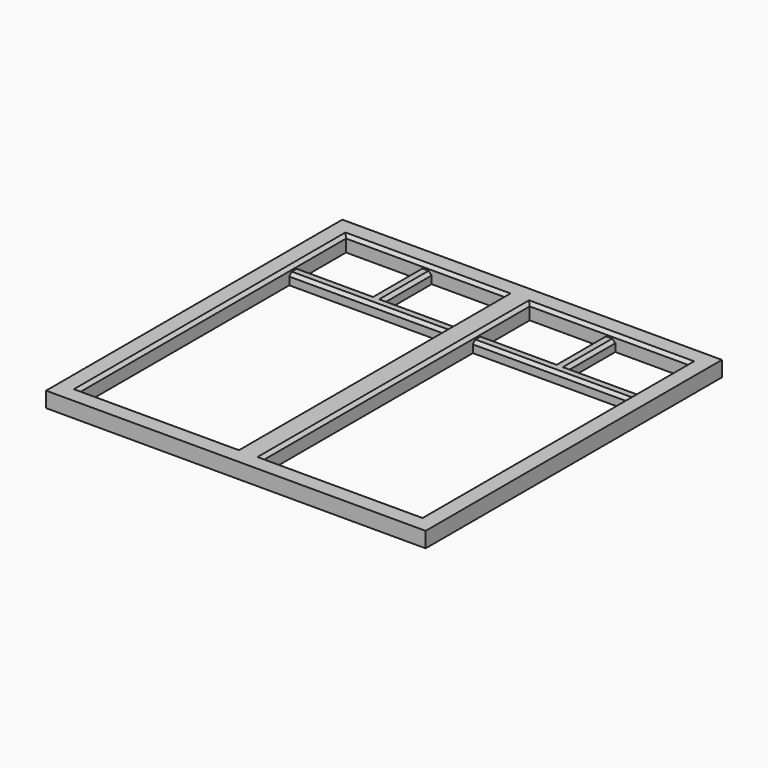
from build123d import *

# Parameters (mm, degrees)
F0_W      = 1230
F0_H      = 1200
F1_DEPTH  = 50
F2_DEPTH  = 35
F3_SIZE   = 10
F3_2_SIZE = 10
F3_3_SIZE = 10


with BuildPart() as f1:
    # F0 (on Top) → F1 (new body)
    with BuildSketch(Plane.XY):
        with Locations((220.3141621128, 45.2047318473)):
            Rectangle(F0_W, F0_H)
        Polygon((-334.6858378872, -494.7952681527), (-334.6858378872, 355.2047318473), (-334.6858378872, 395.2047318473), (-334.6858378872, 585.2047318473), (-97.1858378872, 585.2047318473), (-57.1858378872, 585.2047318473), (180.3141621128, 585.2047318473), (180.3141621128, 395.2047318473), (180.3141621128, 355.2047318473), (180.3141621128, -494.7952681527), align=None, mode=Mode.SUBTRACT)
        Polygon((260.3141621128, -494.7952681527), (260.3141621128, 355.2047318473), (260.3141621128, 395.2047318473), (260.3141621128, 585.2047318473), (497.8141621128, 585.2047318473), (537.8141621128, 585.2047318473), (775.3141621128, 585.2047318473), (775.3141621128, 395.2047318473), (775.3141621128, 355.2047318473), (775.3141621128, -494.7952681527), align=None, mode=Mode.SUBTRACT)
    extrude(amount=F1_DEPTH)

    # F3
    f3_edges = [f1.edges().sort_by_distance(p)[0] for p in [
        (-334.685838, 45.204732, 50),
        (-77.185838, 585.204732, 50),
        (180.314162, 45.204732, 50),
        (260.314162, 45.204732, 50),
        (517.814162, 585.204732, 50),
        (775.314162, 45.204732, 50),
        (517.814162, -494.795268, 50),
        (-77.185838, -494.795268, 50),
    ]]
    chamfer(f3_edges, length=F3_SIZE)


with BuildPart() as f2:
    # F0 (on Top) → F2 (new body)
    with BuildSketch(Plane.XY):
        Polygon((-334.6858378872, 395.2047318473), (-334.6858378872, 355.2047318473), (180.3141621128, 355.2047318473), (180.3141621128, 395.2047318473), (-57.1858378872, 395.2047318473), (-57.1858378872, 585.2047318473), (-97.1858378872, 585.2047318473), (-97.1858378872, 395.2047318473), align=None)
    extrude(amount=F2_DEPTH)

    # F3#2
    f3_2_edges = [f2.edges().sort_by_distance(p)[0] for p in [
        (-77.185838, 355.204732, 35),
        (61.564162, 395.204732, 35),
        (-57.185838, 490.204732, 35),
        (-97.185838, 490.204732, 35),
        (-215.935838, 395.204732, 35),
    ]]
    chamfer(f3_2_edges, length=F3_2_SIZE)


with BuildPart() as f2b:
    # F0 (on Top) → F2, piece 2 (new body)
    with BuildSketch(Plane.XY):
        Polygon((260.3141621128, 395.2047318473), (260.3141621128, 355.2047318473), (775.3141621128, 355.2047318473), (775.3141621128, 395.2047318473), (537.8141621128, 395.2047318473), (537.8141621128, 585.2047318473), (497.8141621128, 585.2047318473), (497.8141621128, 395.2047318473), align=None)
    extrude(amount=F2_DEPTH)

    # F3#3
    f3_3_edges = [f2b.edges().sort_by_distance(p)[0] for p in [
        (517.814162, 355.204732, 35),
        (379.064162, 395.204732, 35),
        (537.814162, 490.204732, 35),
        (656.564162, 395.204732, 35),
        (497.814162, 490.204732, 35),
    ]]
    chamfer(f3_3_edges, length=F3_3_SIZE)


solid = Compound([f1.part, f2.part, f2b.part])
